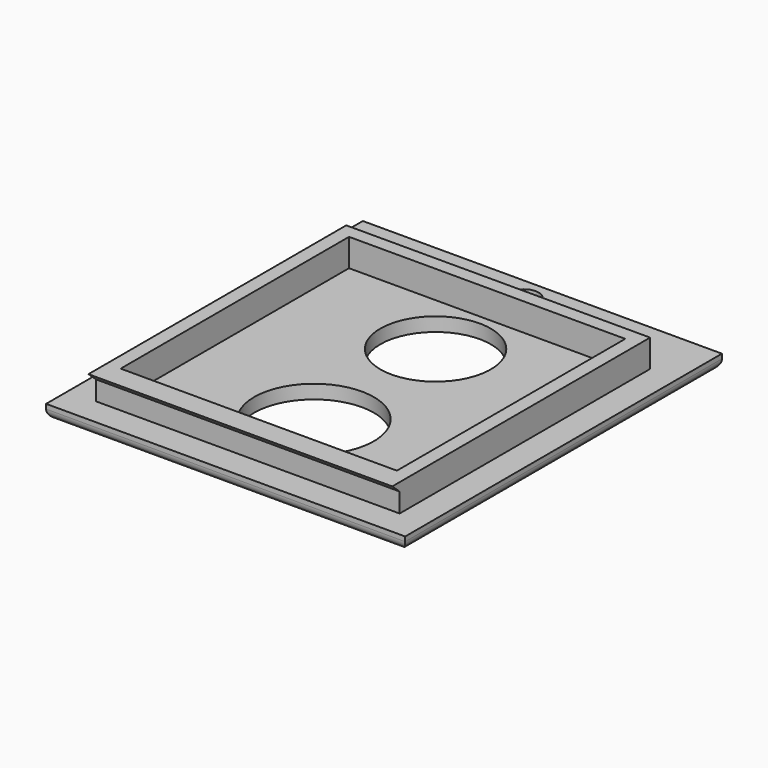
from build123d import *

# Parameters (mm, degrees)
F0_W        = 33
F0_H        = 34
F0_W_2      = 30
F0_H_2      = 31
F1_DEPTH    = 3
F2_W        = 39
F2_H        = 43
F3_DEPTH    = 1.5
F4_D        = 3.2
F5_T1_DEPTH = 44
F5_T3_DEPTH = 48
F7_DEPTH    = 16.5
F8_D        = 12
F9_D        = 13


# Not quite as in the source:
# - a fillet or chamfer that OpenCascade refuses, or shapes differently, is made with other operations: its cross-section is extruded or revolved along the edge and cut away or added


with BuildPart() as f1:
    # F0 (on Top) → F1 (new body)
    with BuildSketch(Plane.XY):
        Rectangle(F0_W, F0_H)
        Rectangle(F0_W_2, F0_H_2, mode=Mode.SUBTRACT)
    extrude(amount=F1_DEPTH)

    # F2 (on Top) → F3 (join)
    with BuildSketch(Plane.XY):
        with Locations((0, 1.5)):
            Rectangle(F2_W, F2_H)
    extrude(amount=-F3_DEPTH)

    # F4 (through all)
    with Locations(Plane.XY):
        with Locations((0, 20.5)):
            Hole(F4_D / 2)

    # F5: fillet of radius 1 on 4 edges, made by hand

    # F5_s2 → F5_t1 (cut)
    with BuildSketch(Plane.YZ.offset(-22)):
        with BuildLine():
            ThreePointArc((23, -0.5), (22.7071067812, -1.2071067812), (22, -1.5))
            Line((22, -1.5), (23, -1.5))
            Line((23, -1.5), (23, -0.5))
        make_face()
        with BuildLine():
            ThreePointArc((-20, -0.5), (-19.7071067812, -1.2071067812), (-19, -1.5))
            Line((-19, -1.5), (-20, -1.5))
            Line((-20, -1.5), (-20, -0.5))
        make_face()
    extrude(amount=F5_T1_DEPTH, mode=Mode.SUBTRACT)

    # F5_s4 → F5_t3 (cut)
    with BuildSketch(Plane.XZ.offset(-25.5)):
        with BuildLine():
            ThreePointArc((-19.5, -0.5), (-19.2071067812, -1.2071067812), (-18.5, -1.5))
            Line((-18.5, -1.5), (-19.5, -1.5))
            Line((-19.5, -1.5), (-19.5, -0.5))
        make_face()
        with BuildLine():
            ThreePointArc((18.5, -1.5), (19.2071067812, -1.2071067812), (19.5, -0.5))
            Line((19.5, -0.5), (19.5, -1.5))
            Line((19.5, -1.5), (18.5, -1.5))
        make_face()
    extrude(amount=F5_T3_DEPTH, mode=Mode.SUBTRACT)

    # F6 (on Right) → F7 (join, symmetric)
    with BuildSketch(Plane.YZ):
        Polygon((-17, 3), (-18, 3), (-17, 2.1), align=None)
    extrude(amount=F7_DEPTH, both=True)

    # F8 (through all)
    with Locations(Plane.XY):
        with Locations((0, 8.5)):
            Hole(F8_D / 2)

    # F9 (through all)
    with Locations(Plane.XY):
        with Locations((0, -8)):
            Hole(F9_D / 2)


solid = f1.part
